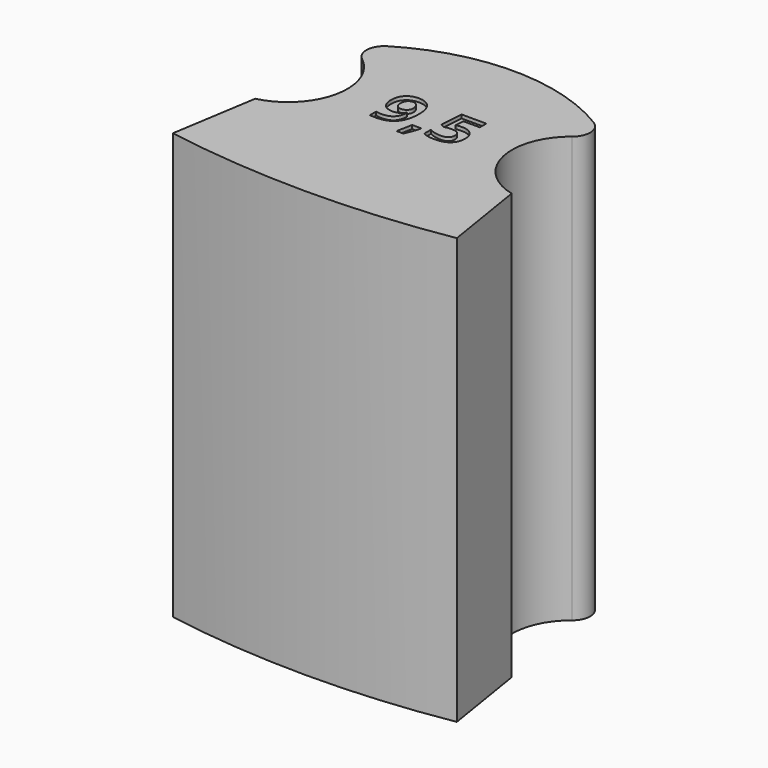
from build123d import *

# Parameters (mm, degrees)
F1_DEPTH     = 120
F2_TEXT_SIZE = 17.9236444334
F3_DEPTH     = 1


# Not quite as in the source:
# - Text() gives the source's letters only with a copy of the font that has no kerning and outlines rounded to 1/6400 em; it was checked with that copy


with BuildPart() as f1:
    # F0 (on Top) → F1 (new body)
    with BuildSketch(Plane.XY):
        with BuildLine():
            Line((3.8687128108, 24.1569802165), (0, 0))
            ThreePointArc((0, 0), (40, -3.356808676), (80, 0))
            Line((80, 0), (76.1312871892, 24.1569802165))
            ThreePointArc((76.1312871892, 24.1569802165), (63.5975554576, 36.8458138953), (69.5972800683, 53.6417728094))
            ThreePointArc((69.5972800683, 53.6417728094), (71.4969098635, 57.8715436357), (69.1043731597, 61.843359684))
            ThreePointArc((69.1043731597, 61.843359684), (40, 70), (10.8956268403, 61.843359684))
            ThreePointArc((10.8956268403, 61.843359684), (8.5030901365, 57.8715436357), (10.4027199317, 53.6417728094))
            ThreePointArc((10.4027199317, 53.6417728094), (16.4024445424, 36.8458138953), (3.8687128108, 24.1569802165))
        make_face()
    extrude(amount=F1_DEPTH)

    # F2 (on face) → F3 (cut)
    with BuildSketch(Plane.XY.offset(120)):
        with Locations((26.9913549386, 33.8757075369)):
            Text('9,5', F2_TEXT_SIZE, font='Open Sans', font_style=FontStyle.BOLD, text_align=(TextAlign.LEFT, TextAlign.BOTTOM))
    extrude(amount=-F3_DEPTH, mode=Mode.SUBTRACT)


solid = f1.part
